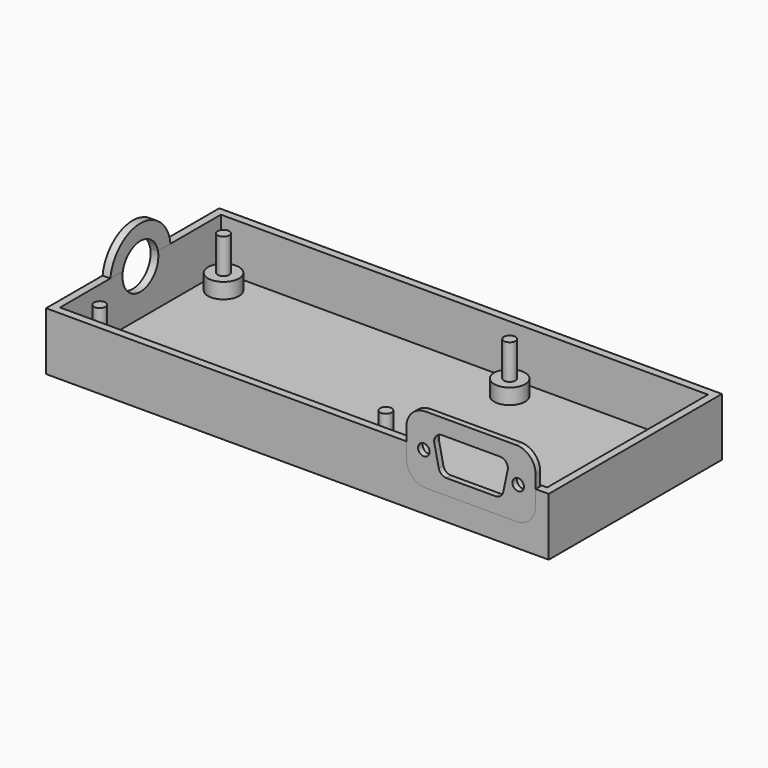
from build123d import *
from build123d import SkipClean  # not in build123d's __all__

# Parameters (mm, degrees)
F0_W      = 130
F0_H      = 56
F1_DEPTH  = 15
F2_T      = -2
F3_R      = 1.5
F4_DEPTH  = 13
F5_R      = 4
F6_DEPTH  = 4
F9_DEPTH  = 5
F7_R      = 1.5
F10_DEPTH = 1.5
F12_DEPTH = 25
F14_DEPTH = 2


with BuildPart() as f1:
    # F0 (on Top) → F1 (new body)
    with BuildSketch(Plane.XY):
        with Locations((65, 28)):
            Rectangle(F0_W, F0_H)
    extrude(amount=F1_DEPTH)

    # F2
    f2_openings = [f1.faces().sort_by_distance(p)[0] for p in [
        (65, 28, 15),
    ]]
    offset(amount=F2_T, openings=f2_openings)

    # F3 (on face) → F4 (join)
    with BuildSketch(Plane.XY.offset(2)):
        with Locations((81.5, 48)):
            Circle(F3_R)
        with Locations((81.5, 8)):
            Circle(F3_R)
        with Locations((7.5, 8)):
            Circle(F3_R)
        with Locations((7.5, 48)):
            Circle(F3_R)
    extrude(amount=F4_DEPTH)

    # F5 (on face) → F6 (join)
    with BuildSketch(Plane.XY.offset(2)):
        with Locations((81.5, 48)):
            Circle(F5_R)
        with Locations((81.5, 8)):
            Circle(F5_R)
        with Locations((7.5, 48)):
            Circle(F5_R)
        with Locations((7.5, 8)):
            Circle(F5_R)
    extrude(amount=F6_DEPTH)

    # F8 (on face) → F9 (cut)
    with BuildSketch(Plane.XZ):
        with BuildLine():
            Line((126.6, 23.4), (93.2, 23.4))
            Line((93.2, 23.4), (93.2, 11))
            ThreePointArc((93.2, 11), (94.6644660941, 7.4644660941), (98.2, 6))
            Line((98.2, 6), (121.6, 6))
            ThreePointArc((121.6, 6), (125.1355339059, 7.4644660941), (126.6, 11))
            Line((126.6, 11), (126.6, 23.4))
        make_face()
    extrude(amount=-F9_DEPTH, mode=Mode.SUBTRACT)

    # F11 (on face) → F12 (cut)
    with BuildSketch(Plane(origin=(0, 0, 0), x_dir=(0, -1, 0), z_dir=(-1, 0, 0))):
        with BuildLine():
            ThreePointArc((-33.6745043836, 15), (-28.6032721504, 8.0314592216), (-22.2, 13.8))
            ThreePointArc((-22.2, 13.8), (-22.2314592216, 14.4032721504), (-22.3254956164, 15))
            Line((-22.3254956164, 15), (-33.6745043836, 15))
        make_face()
    extrude(amount=-F12_DEPTH, mode=Mode.SUBTRACT)

    # F13 (on face) → F14 (join)
    with BuildSketch(Plane(origin=(0, 0, 0), x_dir=(0, -1, 0), z_dir=(-1, 0, 0))):
        with BuildLine():
            ThreePointArc((-33.6745043836, 15), (-28, 19.6), (-22.3254956164, 15))
            Line((-22.3254956164, 15), (-18.2737468674, 15))
            ThreePointArc((-18.2737468674, 15), (-28, 23.6), (-37.7262531326, 15))
            Line((-37.7262531326, 15), (-33.6745043836, 15))
        make_face()
    with SkipClean():  # cleaning this boolean's faces spoils the solid; the shape is the same uncleaned
        extrude(amount=-F14_DEPTH)


with BuildPart() as f10:
    # F7 (on face) → F10 (new body)
    with BuildSketch(Plane.XZ):
        with BuildLine():
            Line((121.6, 23.4), (98.2, 23.4))
            ThreePointArc((98.2, 23.4), (94.6644660941, 21.9355339059), (93.2, 18.4))
            Line((93.2, 18.4), (93.2, 11))
            ThreePointArc((93.2, 11), (94.6644660941, 7.4644660941), (98.2, 6))
            Line((98.2, 6), (121.6, 6))
            ThreePointArc((121.6, 6), (125.1355339059, 7.4644660941), (126.6, 11))
            Line((126.6, 11), (126.6, 18.4))
            ThreePointArc((126.6, 18.4), (125.1355339059, 21.9355339059), (121.6, 23.4))
        make_face()
        with Locations((97.7, 14.5323744416)):
            Circle(F7_R, mode=Mode.SUBTRACT)
        with Locations((122.1, 14.5323744416)):
            Circle(F7_R, mode=Mode.SUBTRACT)
        with BuildLine():
            ThreePointArc((100.413788142, 16.9837847111), (100.8155820096, 18.6584850858), (102.37, 19.4))
            Line((102.37, 19.4), (117.4293995654, 19.4))
            ThreePointArc((117.4293995654, 19.4), (118.9838175558, 18.6584850858), (119.3856114233, 16.9837847111))
            Line((119.3856114233, 16.9837847111), (118.2366752531, 11.5837847111))
            ThreePointArc((118.2366752531, 11.5837847111), (117.5389484809, 10.4455820096), (116.2804633952, 10))
            Line((116.2804633952, 10), (103.5189361702, 10))
            ThreePointArc((103.5189361702, 10), (102.2604510845, 10.4455820096), (101.5627243122, 11.5837847111))
            Line((101.5627243122, 11.5837847111), (100.413788142, 16.9837847111))
        make_face(mode=Mode.SUBTRACT)
    extrude(amount=-F10_DEPTH)


solid = Compound([f1.part, f10.part])
